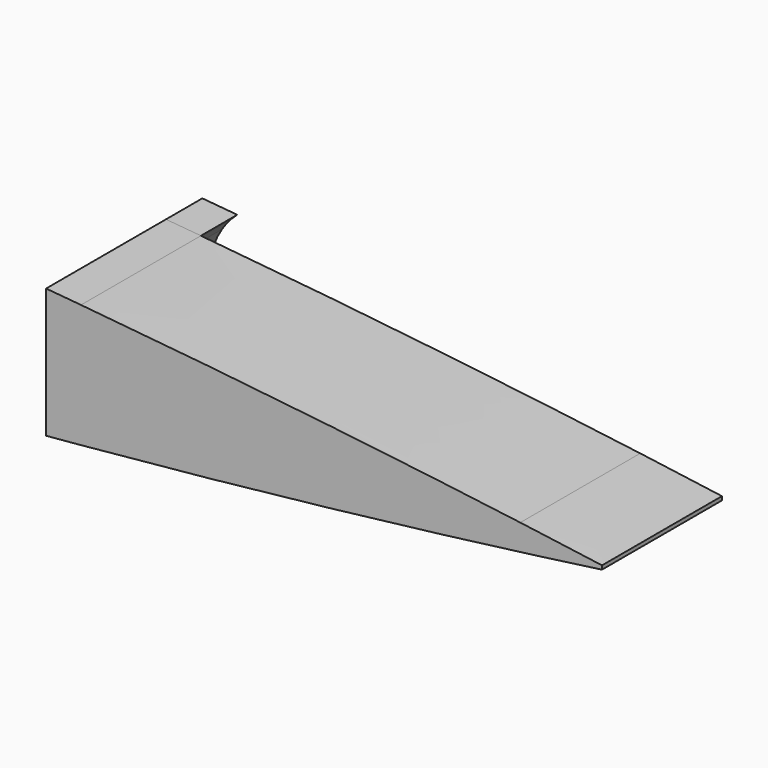
from build123d import *

# Parameters (mm, degrees)
F1_DEPTH = 82.5
F2_DEPTH = 25
F3_R     = 12.5
F4_DEPTH = 60


with BuildPart() as f1:
    # F0 (on Front) → F1 (new body)
    with BuildSketch(Plane.XZ):
        with BuildLine():
            add(Edge.make_bspline(
                [(524.024, 35.6715651167), (530.4529675183, 35.1109062879), (536.8603422789, 34.540475321), (543.2421, 33.9614)],
                knots=[0.6159550767, 0.6159550767, 0.6159550767, 0.6159550767, 0.635369827, 0.635369827, 0.635369827, 0.635369827], degree=3))
            Line((524.024, 35.6715651167), (524.024, 25.1107127602))
            add(Edge.make_bspline(
                [(524.024, 25.1107127602), (526.6770638269, 24.868020166), (530.2603237936, 24.5375720807), (533.8432643328, 24.2037227591), (534.7735361573, 24.1168150682)],
                knots=[513.3651484855, 513.3651484855, 513.3651484855, 513.3651484855, 521.3575419642, 524.1605032173, 524.1605032173, 524.1605032173, 524.1605032173], degree=3))
            ThreePointArc((534.7735361573, 24.1168150682), (538.650838246, 29.3461907199), (543.2421, 33.9614))
        make_face()
        with BuildLine():
            Line((524.024, -23.2286070743), (524.024, -35.6715651167))
            add(Edge.make_bspline(
                [(524.024, -35.6715651167), (530.4529675183, -35.1109062879), (536.8603422789, -34.540475321), (543.2421, -33.9614)],
                knots=[0.6159550767, 0.6159550767, 0.6159550767, 0.6159550767, 0.635369827, 0.635369827, 0.635369827, 0.635369827], degree=3))
            ThreePointArc((543.2421, -33.9614), (537.9689313182, -28.5343309954), (533.6796750092, -22.3004184004))
            add(Edge.make_bspline(
                [(524.024, -23.2286070743), (526.7063477836, -22.9731340758), (529.9249490386, -22.6641634275), (533.1432820941, -22.3524476401), (533.6796750092, -22.3004184004)],
                knots=[513.2741132252, 513.2741132252, 513.2741132252, 513.2741132252, 521.3575419641, 522.9742691651, 522.9742691651, 522.9742691651, 522.9742691651], degree=3))
        make_face()
        with BuildLine():
            add(Edge.make_bspline(
                [(524.024, 25.1107127602), (526.6770638269, 24.868020166), (530.2603237936, 24.5375720807), (533.8432643328, 24.2037227591), (534.7735361573, 24.1168150682)],
                knots=[513.3651484855, 513.3651484855, 513.3651484855, 513.3651484855, 521.3575419642, 524.1605032173, 524.1605032173, 524.1605032173, 524.1605032173], degree=3))
            Line((524.024, 25.1107127602), (524.024, 0))
            Line((524.024, 0), (527.7653672657, 0))
            ThreePointArc((527.7653672657, 0), (529.5529130431, 12.5572210326), (534.7735361573, 24.1168150682))
        make_face()
        with BuildLine():
            Line((524.024, 0), (524.024, -23.2286070743))
            add(Edge.make_bspline(
                [(524.024, -23.2286070743), (526.7063477836, -22.9731340758), (529.9249490386, -22.6641634275), (533.1432820941, -22.3524476401), (533.6796750092, -22.3004184004)],
                knots=[513.2741132252, 513.2741132252, 513.2741132252, 513.2741132252, 521.3575419641, 522.9742691651, 522.9742691651, 522.9742691651, 522.9742691651], degree=3))
            ThreePointArc((533.6796750092, -22.3004184004), (529.2690677016, -11.535680484), (527.7653672657, 0))
            Line((527.7653672657, 0), (524.024, 0))
        make_face()
        with BuildLine():
            add(Edge.make_bspline(
                [(543.2421, 33.9614), (549.5750436875, 33.3867540232), (562.1338476881, 32.225672374), (580.7053749717, 30.4486309004), (598.8899905971, 28.6520916952), (616.645063933, 26.8456524154), (633.9293517992, 25.0378311486), (650.7021084927, 23.2377895738), (666.924523511, 21.4542053534), (682.5583919944, 19.6948931431), (697.5675188661, 17.9689901739), (711.9166403588, 16.2843520174), (725.5723159977, 14.6495448382), (738.5025922877, 13.0722198932), (750.6773575973, 11.5611505206), (762.0679980169, 10.123355488), (772.6482697775, 8.767506964), (780.1684058461, 7.7893010713), (784.1801262556, 7.2631536294), (785.0296548206, 7.1515377434)],
                knots=[0.635369827, 0.635369827, 0.635369827, 0.635369827, 0.654636074, 0.6737293504, 0.6926255053, 0.7112999065, 0.7297277282, 0.747883428, 0.7657412837, 0.7832747177, 0.8004566202, 0.8172588362, 0.8336522425, 0.8496064603, 0.8650895564, 0.8800677295, 0.8945049966, 0.9083621399, 0.9121165786, 0.9121165786, 0.9121165786, 0.9121165786], degree=3))
            ThreePointArc((543.2421, 33.9614), (538.650838246, 29.3461907199), (534.7735361573, 24.1168150682))
            add(Edge.make_bspline(
                [(534.7735361573, 24.1168150682), (547.4888491387, 22.9289273345), (570.2810474133, 20.7234876988), (602.9514797769, 17.4132456465), (629.5721727855, 14.5753690345), (646.1150179567, 12.7470797563), (652.7777391491, 12)],
                knots=[524.1605032173, 524.1605032173, 524.1605032173, 524.1605032173, 562.4724553443, 592.8561025481, 622.6732889332, 642.7866986571, 642.7866986571, 642.7866986571, 642.7866986571], degree=3))
            Line((652.7777391491, 12), (665.973, 12))
            ThreePointArc((665.973, 12), (669.6925428199, 11.4089877382), (673.0457030707, 9.6941668684))
            add(Edge.make_bspline(
                [(673.0457030707, 9.6941668684), (678.6430527256, 9.0482316549), (693.2761814168, 7.3399638663), (715.1021603081, 4.7178028299), (732.4511827497, 2.5525104658), (740.7700852943, 1.4970109313), (741.8962423005, 1.3538186415)],
                knots=[663.1854009899, 663.1854009899, 663.1854009899, 663.1854009899, 680.0888797975, 707.3828314911, 729.1339381861, 732.5396092821, 732.5396092821, 732.5396092821, 732.5396092821], degree=3))
            add(Edge.make_bspline(
                [(741.8962423005, 1.3538186415), (746.2843670673, 1.9285048035), (754.6747553371, 3.0362373869), (766.9194584147, 4.6744667559), (776.9091256945, 6.0324501077), (782.8966080674, 6.8566568424), (785.0296548206, 7.1515377434)],
                knots=[732.5396092819, 732.5396092819, 732.5396092819, 732.5396092819, 745.8163943039, 757.9291810967, 769.6010098164, 776.0610078587, 776.0610078587, 776.0610078587, 776.0610078587], degree=3))
        make_face()
        with BuildLine():
            ThreePointArc((533.6796750092, -22.3004184004), (537.9689313182, -28.5343309954), (543.2421, -33.9614))
            add(Edge.make_bspline(
                [(543.2421, -33.9614), (549.5750436875, -33.3867540232), (562.1338476881, -32.225672374), (580.7053749717, -30.4486309004), (598.8899905971, -28.6520916952), (616.645063933, -26.8456524154), (633.9293517992, -25.0378311486), (650.7021084927, -23.2377895738), (666.924523511, -21.4542053534), (682.5583919944, -19.6948931431), (697.5675188661, -17.9689901739), (711.9166403588, -16.2843520174), (725.5723159977, -14.6495448382), (738.5025922877, -13.0722198932), (750.6773575973, -11.5611505206), (762.0679980169, -10.123355488), (772.6482697775, -8.767506964), (782.3928967751, -7.4999432572), (789.9922436278, -6.4986676858), (794.3093421293, -5.9243671687), (795.7553403022, -5.731408495)],
                knots=[0.635369827, 0.635369827, 0.635369827, 0.635369827, 0.654636074, 0.6737293504, 0.6926255053, 0.7112999065, 0.7297277282, 0.747883428, 0.7657412837, 0.7832747177, 0.8004566202, 0.8172588362, 0.8336522425, 0.8496064603, 0.8650895564, 0.8800677295, 0.8945049966, 0.9083621399, 0.921596776, 0.9284158886, 0.9284158886, 0.9284158886, 0.9284158886], degree=3))
            add(Edge.make_bspline(
                [(752.4752127939, 0), (753.3385987131, -0.1111737387), (758.2064040588, -0.7388852768), (766.9317355754, -1.8729638235), (778.4845581837, -3.3993366737), (788.0433504555, -4.682906586), (793.7449819172, -5.4572465403), (795.7553403022, -5.731408495)],
                knots=[743.2048524915, 743.2048524915, 743.2048524915, 743.2048524915, 745.816394304, 757.9291810969, 769.6010098166, 780.7760242539, 786.8629233002, 786.8629233002, 786.8629233002, 786.8629233002], degree=3))
            Line((752.4752127939, 0), (731.4902537549, 0))
            add(Edge.make_bspline(
                [(675.7749550869, -6.922548409), (680.4704196169, -6.3608211123), (694.1976504575, -4.7032327955), (712.7702276209, -2.4012449385), (726.6428498764, -0.6263462539), (731.4902537549, 0)],
                knots=[665.902054437, 665.902054437, 665.902054437, 665.902054437, 680.0888797974, 707.382831491, 722.0459285975, 722.0459285975, 722.0459285975, 722.0459285975], degree=3))
            ThreePointArc((675.7749550869, -6.922548409), (671.4924845363, -10.6552940107), (665.973, -12))
            Line((665.973, -12), (632.0462382215, -12))
            add(Edge.make_bspline(
                [(579.5327593007, -17.6845550908), (587.4225464727, -16.8640224682), (604.9318542045, -15.0134548613), (622.4325289508, -13.08262656), (632.0462382215, -12)],
                knots=[569.0591158558, 569.0591158558, 569.0591158558, 569.0591158558, 592.856102548, 621.8794937898, 621.8794937898, 621.8794937898, 621.8794937898], degree=3))
            add(Edge.make_bspline(
                [(569.024, -20), (574.601223494, -20), (579.5327593007, -17.6845550908)],
                knots=[4.7123889804, 4.7123889804, 4.7123889804, 5.1983473252, 5.1983473252, 5.1983473252], degree=2, weights=[1, 0.9706255083, 1]))
            add(Edge.make_bspline(
                [(563.3375761456, -19.3507371729), (566.1338768344, -20), (569.024, -20)],
                knots=[4.4568882152, 4.4568882152, 4.4568882152, 4.7123889804, 4.7123889804, 4.7123889804], degree=2, weights=[1, 0.9918510117, 1]))
            add(Edge.make_bspline(
                [(533.6796750092, -22.3004184004), (543.5680241797, -21.3412646258), (553.4538623678, -20.3564530629), (563.3375761456, -19.3507371729)],
                knots=[522.9742691651, 522.9742691651, 522.9742691651, 522.9742691651, 552.7784716909, 552.7784716909, 552.7784716909, 552.7784716909], degree=3))
        make_face()
        with BuildLine():
            add(Edge.make_bspline(
                [(534.7735361573, 24.1168150682), (547.4888491387, 22.9289273345), (570.2810474133, 20.7234876988), (602.9514797769, 17.4132456465), (629.5721727855, 14.5753690345), (646.1150179567, 12.7470797563), (652.7777391491, 12)],
                knots=[524.1605032173, 524.1605032173, 524.1605032173, 524.1605032173, 562.4724553443, 592.8561025481, 622.6732889332, 642.7866986571, 642.7866986571, 642.7866986571, 642.7866986571], degree=3))
            ThreePointArc((534.7735361573, 24.1168150682), (529.5529130431, 12.5572210326), (527.7653672657, 0))
            Line((527.7653672657, 0), (546.524, 0))
            add(Edge.make_bspline(
                [(591.524, 0), (591.524, 20), (569.024, 20), (546.524, 20), (546.524, 0)],
                knots=[0, 0, 0, 1.5707963268, 1.5707963268, 3.1415926536, 3.1415926536, 3.1415926536], degree=2, weights=[1, 0.7071067812, 1, 0.7071067812, 1]))
            Line((591.524, 0), (623.973, 0))
            Line((623.973, 0), (623.973, 10))
            ThreePointArc((623.973, 10), (624.5587864376, 11.4142135624), (625.973, 12))
            Line((625.973, 12), (652.7777391491, 12))
        make_face()
        with BuildLine():
            ThreePointArc((527.7653672657, 0), (529.2690677016, -11.535680484), (533.6796750092, -22.3004184004))
            add(Edge.make_bspline(
                [(533.6796750092, -22.3004184004), (543.5680241797, -21.3412646258), (553.4538623678, -20.3564530629), (563.3375761456, -19.3507371729)],
                knots=[522.9742691651, 522.9742691651, 522.9742691651, 522.9742691651, 552.7784716909, 552.7784716909, 552.7784716909, 552.7784716909], degree=3))
            add(Edge.make_bspline(
                [(546.524, 0), (546.524, -15.4468544374), (563.3375761456, -19.3507371729)],
                knots=[3.1415926536, 3.1415926536, 3.1415926536, 4.4568882152, 4.4568882152, 4.4568882152], degree=2, weights=[1, 0.7914322299, 1]))
            Line((546.524, 0), (527.7653672657, 0))
        make_face()
        with BuildLine():
            add(Edge.make_bspline(
                [(785.0296548206, 7.1515377434), (787.174768668, 6.8697005072), (792.0785180819, 6.2224623401), (799.2875794028, 5.2606805783), (806.398007937, 4.3017234095), (812.5937368846, 3.4579115596), (817.8623783077, 2.7342517017), (822.1845332462, 2.1365671069), (825.5717903187, 1.6654782983), (827.9484571682, 1.33323589), (829.4727060537, 1.1198422864), (829.8586880275, 1.0656429389), (830, 1.0458)],
                knots=[0.9121165786, 0.9121165786, 0.9121165786, 0.9121165786, 0.921596776, 0.9341612481, 0.9460018444, 0.9570561288, 0.9672492741, 0.9764880356, 0.9846490394, 0.9915545746, 0.9969080429, 1, 1, 1, 1], degree=3))
            add(Edge.make_bspline(
                [(741.8962423005, 1.3538186415), (746.2843670673, 1.9285048035), (754.6747553371, 3.0362373869), (766.9194584147, 4.6744667559), (776.9091256945, 6.0324501077), (782.8966080674, 6.8566568424), (785.0296548206, 7.1515377434)],
                knots=[732.5396092819, 732.5396092819, 732.5396092819, 732.5396092819, 745.8163943039, 757.9291810967, 769.6010098164, 776.0610078587, 776.0610078587, 776.0610078587, 776.0610078587], degree=3))
            add(Edge.make_bspline(
                [(741.8962423005, 1.3538186415), (745.4229300003, 0.9053958333), (748.9492417496, 0.4540210524), (752.4752127939, 0)],
                knots=[732.5396092821, 732.5396092821, 732.5396092821, 732.5396092821, 743.2048524915, 743.2048524915, 743.2048524915, 743.2048524915], degree=3))
            Line((752.4752127939, 0), (830, 0))
            Line((830, 0), (830, 1.0458))
        make_face()
        with BuildLine():
            add(Edge.make_bspline(
                [(752.4752127939, 0), (753.3385987131, -0.1111737387), (758.2064040588, -0.7388852768), (766.9317355754, -1.8729638235), (778.4845581837, -3.3993366737), (788.0433504555, -4.682906586), (793.7449819172, -5.4572465403), (795.7553403022, -5.731408495)],
                knots=[743.2048524915, 743.2048524915, 743.2048524915, 743.2048524915, 745.816394304, 757.9291810969, 769.6010098166, 780.7760242539, 786.8629233002, 786.8629233002, 786.8629233002, 786.8629233002], degree=3))
            add(Edge.make_bspline(
                [(795.7553403022, -5.731408495), (796.9736482838, -5.568833537), (800.6549707765, -5.0762655667), (806.398007937, -4.3017234095), (812.5937368846, -3.4579115596), (817.8623783077, -2.7342517017), (822.1845332462, -2.1365671069), (825.5717903187, -1.6654782983), (827.9484571682, -1.33323589), (829.4727060537, -1.1198422864), (829.8586880275, -1.0656429389), (830, -1.0458)],
                knots=[0.9284158886, 0.9284158886, 0.9284158886, 0.9284158886, 0.9341612481, 0.9460018444, 0.9570561288, 0.9672492741, 0.9764880356, 0.9846490394, 0.9915545746, 0.9969080429, 1, 1, 1, 1], degree=3))
            Line((830, -1.0458), (830, 0))
            Line((830, 0), (752.4752127939, 0))
        make_face()
        with BuildLine():
            Line((665.973, 12), (652.7777391491, 12))
            add(Edge.make_bspline(
                [(652.7777391491, 12), (655.762922623, 11.6652763822), (660.161514663, 11.1688961032), (664.5595773708, 10.6678568096), (665.973, 10.5063520034)],
                knots=[642.7866986571, 642.7866986571, 642.7866986571, 642.7866986571, 651.7983646979, 656.0662217526, 656.0662217526, 656.0662217526, 656.0662217526], degree=3))
            Line((665.973, 10.5063520034), (665.973, 12))
        make_face()
        with BuildLine():
            add(Edge.make_bspline(
                [(652.7777391491, 12), (655.762922623, 11.6652763822), (660.161514663, 11.1688961032), (664.5595773708, 10.6678568096), (665.973, 10.5063520034)],
                knots=[642.7866986571, 642.7866986571, 642.7866986571, 642.7866986571, 651.7983646979, 656.0662217526, 656.0662217526, 656.0662217526, 656.0662217526], degree=3))
            Line((652.7777391491, 12), (625.973, 12))
            ThreePointArc((625.973, 12), (624.5587864376, 11.4142135624), (623.973, 10))
            Line((623.973, 10), (623.973, 0))
            Line((623.973, 0), (665.973, 0))
            Line((665.973, 0), (665.973, 10.5063520034))
        make_face()
        with BuildLine():
            add(Edge.make_bspline(
                [(546.524, 0), (546.524, -15.4468544374), (563.3375761456, -19.3507371729)],
                knots=[3.1415926536, 3.1415926536, 3.1415926536, 4.4568882152, 4.4568882152, 4.4568882152], degree=2, weights=[1, 0.7914322299, 1]))
            add(Edge.make_bspline(
                [(563.3375761456, -19.3507371729), (566.5523093603, -19.0236224518), (571.9509432397, -18.4705327095), (577.3489807289, -17.911666611), (579.5327593007, -17.6845550908)],
                knots=[552.7784716909, 552.7784716909, 552.7784716909, 552.7784716909, 562.4724553442, 569.0591158558, 569.0591158558, 569.0591158558, 569.0591158558], degree=3))
            add(Edge.make_bspline(
                [(579.5327593007, -17.6845550908), (591.524, -12.0544515447), (591.524, 0)],
                knots=[5.1983473252, 5.1983473252, 5.1983473252, 6.2831853072, 6.2831853072, 6.2831853072], degree=2, weights=[1, 0.8564624828, 1]))
            Line((591.524, 0), (546.524, 0))
        make_face()
        with BuildLine():
            add(Edge.make_bspline(
                [(563.3375761456, -19.3507371729), (566.5523093603, -19.0236224518), (571.9509432397, -18.4705327095), (577.3489807289, -17.911666611), (579.5327593007, -17.6845550908)],
                knots=[552.7784716909, 552.7784716909, 552.7784716909, 552.7784716909, 562.4724553442, 569.0591158558, 569.0591158558, 569.0591158558, 569.0591158558], degree=3))
            add(Edge.make_bspline(
                [(563.3375761456, -19.3507371729), (566.1338768344, -20), (569.024, -20)],
                knots=[4.4568882152, 4.4568882152, 4.4568882152, 4.7123889804, 4.7123889804, 4.7123889804], degree=2, weights=[1, 0.9918510117, 1]))
            add(Edge.make_bspline(
                [(569.024, -20), (574.601223494, -20), (579.5327593007, -17.6845550908)],
                knots=[4.7123889804, 4.7123889804, 4.7123889804, 5.1983473252, 5.1983473252, 5.1983473252], degree=2, weights=[1, 0.9706255083, 1]))
        make_face()
        with BuildLine():
            add(Edge.make_bspline(
                [(731.4902537549, 0), (733.8334453003, 0.3027701597), (737.3022307159, 0.7531116765), (740.7706302145, 1.2064040341), (741.8962423005, 1.3538186415)],
                knots=[722.0459285975, 722.0459285975, 722.0459285975, 722.0459285975, 729.1339381859, 732.5396092819, 732.5396092819, 732.5396092819, 732.5396092819], degree=3))
            add(Edge.make_bspline(
                [(673.0457030707, 9.6941668684), (678.6430527256, 9.0482316549), (693.2761814168, 7.3399638663), (715.1021603081, 4.7178028299), (732.4511827497, 2.5525104658), (740.7700852943, 1.4970109313), (741.8962423005, 1.3538186415)],
                knots=[663.1854009899, 663.1854009899, 663.1854009899, 663.1854009899, 680.0888797975, 707.3828314911, 729.1339381861, 732.5396092821, 732.5396092821, 732.5396092821, 732.5396092821], degree=3))
            ThreePointArc((673.0457030707, 9.6941668684), (676.6704865471, 5.4372586453), (677.973, 0))
            Line((677.973, 0), (731.4902537549, 0))
        make_face()
        with BuildLine():
            add(Edge.make_bspline(
                [(741.8962423005, 1.3538186415), (745.4229300003, 0.9053958333), (748.9492417496, 0.4540210524), (752.4752127939, 0)],
                knots=[732.5396092821, 732.5396092821, 732.5396092821, 732.5396092821, 743.2048524915, 743.2048524915, 743.2048524915, 743.2048524915], degree=3))
            add(Edge.make_bspline(
                [(731.4902537549, 0), (733.8334453003, 0.3027701597), (737.3022307159, 0.7531116765), (740.7706302145, 1.2064040341), (741.8962423005, 1.3538186415)],
                knots=[722.0459285975, 722.0459285975, 722.0459285975, 722.0459285975, 729.1339381859, 732.5396092819, 732.5396092819, 732.5396092819, 732.5396092819], degree=3))
            Line((731.4902537549, 0), (752.4752127939, 0))
        make_face()
        with BuildLine():
            add(Edge.make_bspline(
                [(591.524, 0), (591.524, 20), (569.024, 20), (546.524, 20), (546.524, 0)],
                knots=[0, 0, 0, 1.5707963268, 1.5707963268, 3.1415926536, 3.1415926536, 3.1415926536], degree=2, weights=[1, 0.7071067812, 1, 0.7071067812, 1]))
            Line((546.524, 0), (591.524, 0))
        make_face()
        with BuildLine():
            Line((665.973, 12), (665.973, 10.5063520034))
            add(Edge.make_bspline(
                [(665.973, 10.5063520034), (668.3307193205, 10.2369470894), (670.6882868311, 9.9662131504), (673.0457030707, 9.6941668684)],
                knots=[656.0662217526, 656.0662217526, 656.0662217526, 656.0662217526, 663.1854009899, 663.1854009899, 663.1854009899, 663.1854009899], degree=3))
            ThreePointArc((673.0457030707, 9.6941668684), (669.6925428199, 11.4089877382), (665.973, 12))
        make_face()
        with BuildLine():
            add(Edge.make_bspline(
                [(665.973, 10.5063520034), (668.3307193205, 10.2369470894), (670.6882868311, 9.9662131504), (673.0457030707, 9.6941668684)],
                knots=[656.0662217526, 656.0662217526, 656.0662217526, 656.0662217526, 663.1854009899, 663.1854009899, 663.1854009899, 663.1854009899], degree=3))
            Line((665.973, 10.5063520034), (665.973, 0))
            Line((665.973, 0), (677.973, 0))
            ThreePointArc((677.973, 0), (676.6704865471, 5.4372586453), (673.0457030707, 9.6941668684))
        make_face()
        with BuildLine():
            add(Edge.make_bspline(
                [(579.5327593007, -17.6845550908), (591.524, -12.0544515447), (591.524, 0)],
                knots=[5.1983473252, 5.1983473252, 5.1983473252, 6.2831853072, 6.2831853072, 6.2831853072], degree=2, weights=[1, 0.8564624828, 1]))
            add(Edge.make_bspline(
                [(579.5327593007, -17.6845550908), (587.4225464727, -16.8640224682), (604.9318542045, -15.0134548613), (622.4325289508, -13.08262656), (632.0462382215, -12)],
                knots=[569.0591158558, 569.0591158558, 569.0591158558, 569.0591158558, 592.856102548, 621.8794937898, 621.8794937898, 621.8794937898, 621.8794937898], degree=3))
            Line((632.0462382215, -12), (625.973, -12))
            ThreePointArc((625.973, -12), (624.5587864376, -11.4142135624), (623.973, -10))
            Line((623.973, -10), (623.973, 0))
            Line((623.973, 0), (591.524, 0))
        make_face()
        with BuildLine():
            add(Edge.make_bspline(
                [(675.7749550869, -6.922548409), (680.4704196169, -6.3608211123), (694.1976504575, -4.7032327955), (712.7702276209, -2.4012449385), (726.6428498764, -0.6263462539), (731.4902537549, 0)],
                knots=[665.902054437, 665.902054437, 665.902054437, 665.902054437, 680.0888797974, 707.382831491, 722.0459285975, 722.0459285975, 722.0459285975, 722.0459285975], degree=3))
            Line((731.4902537549, 0), (677.973, 0))
            ThreePointArc((677.973, 0), (677.4102955947, -3.6315657062), (675.7749550869, -6.922548409))
        make_face()
        with BuildLine():
            Line((665.973, -8.0874938306), (665.973, 0))
            Line((665.973, 0), (623.973, 0))
            Line((623.973, 0), (623.973, -10))
            ThreePointArc((623.973, -10), (624.5587864376, -11.4142135624), (625.973, -12))
            Line((625.973, -12), (632.0462382215, -12))
            add(Edge.make_bspline(
                [(632.0462382215, -12), (632.3091749564, -11.9703899624), (642.2194339984, -10.8537488755), (653.528780869, -9.5529086768), (664.5718113348, -8.2529185042), (665.973, -8.0874938306)],
                knots=[621.8794937898, 621.8794937898, 621.8794937898, 621.8794937898, 622.6732889331, 651.7983646977, 656.0311218622, 656.0311218622, 656.0311218622, 656.0311218622], degree=3))
        make_face()
        with BuildLine():
            Line((677.973, 0), (665.973, 0))
            Line((665.973, 0), (665.973, -8.0874938306))
            add(Edge.make_bspline(
                [(665.973, -8.0874938306), (669.2406192612, -7.7017179081), (672.5079370891, -7.3133879471), (675.7749550869, -6.922548409)],
                knots=[656.0311218622, 656.0311218622, 656.0311218622, 656.0311218622, 665.902054437, 665.902054437, 665.902054437, 665.902054437], degree=3))
            ThreePointArc((675.7749550869, -6.922548409), (677.4102955947, -3.6315657062), (677.973, 0))
        make_face()
        with BuildLine():
            add(Edge.make_bspline(
                [(632.0462382215, -12), (632.3091749564, -11.9703899624), (642.2194339984, -10.8537488755), (653.528780869, -9.5529086768), (664.5718113348, -8.2529185042), (665.973, -8.0874938306)],
                knots=[621.8794937898, 621.8794937898, 621.8794937898, 621.8794937898, 622.6732889331, 651.7983646977, 656.0311218622, 656.0311218622, 656.0311218622, 656.0311218622], degree=3))
            Line((632.0462382215, -12), (665.973, -12))
            Line((665.973, -12), (665.973, -8.0874938306))
        make_face()
        with BuildLine():
            ThreePointArc((665.973, -12), (671.4924845363, -10.6552940107), (675.7749550869, -6.922548409))
            add(Edge.make_bspline(
                [(665.973, -8.0874938306), (669.2406192612, -7.7017179081), (672.5079370891, -7.3133879471), (675.7749550869, -6.922548409)],
                knots=[656.0311218622, 656.0311218622, 656.0311218622, 656.0311218622, 665.902054437, 665.902054437, 665.902054437, 665.902054437], degree=3))
            Line((665.973, -8.0874938306), (665.973, -12))
        make_face()
    extrude(amount=F1_DEPTH)

    # F0 (on Front) → F2 (join)
    with BuildSketch(Plane.XZ):
        with BuildLine():
            add(Edge.make_bspline(
                [(524.024, 35.6715651167), (530.4529675183, 35.1109062879), (536.8603422789, 34.540475321), (543.2421, 33.9614)],
                knots=[0.6159550767, 0.6159550767, 0.6159550767, 0.6159550767, 0.635369827, 0.635369827, 0.635369827, 0.635369827], degree=3))
            Line((524.024, 35.6715651167), (524.024, 25.1107127602))
            add(Edge.make_bspline(
                [(524.024, 25.1107127602), (526.6770638269, 24.868020166), (530.2603237936, 24.5375720807), (533.8432643328, 24.2037227591), (534.7735361573, 24.1168150682)],
                knots=[513.3651484855, 513.3651484855, 513.3651484855, 513.3651484855, 521.3575419642, 524.1605032173, 524.1605032173, 524.1605032173, 524.1605032173], degree=3))
            ThreePointArc((534.7735361573, 24.1168150682), (538.650838246, 29.3461907199), (543.2421, 33.9614))
        make_face()
        with BuildLine():
            Line((524.024, -23.2286070743), (524.024, -35.6715651167))
            add(Edge.make_bspline(
                [(524.024, -35.6715651167), (530.4529675183, -35.1109062879), (536.8603422789, -34.540475321), (543.2421, -33.9614)],
                knots=[0.6159550767, 0.6159550767, 0.6159550767, 0.6159550767, 0.635369827, 0.635369827, 0.635369827, 0.635369827], degree=3))
            ThreePointArc((543.2421, -33.9614), (537.9689313182, -28.5343309954), (533.6796750092, -22.3004184004))
            add(Edge.make_bspline(
                [(524.024, -23.2286070743), (526.7063477836, -22.9731340758), (529.9249490386, -22.6641634275), (533.1432820941, -22.3524476401), (533.6796750092, -22.3004184004)],
                knots=[513.2741132252, 513.2741132252, 513.2741132252, 513.2741132252, 521.3575419641, 522.9742691651, 522.9742691651, 522.9742691651, 522.9742691651], degree=3))
        make_face()
        with BuildLine():
            add(Edge.make_bspline(
                [(524.024, 25.1107127602), (526.6770638269, 24.868020166), (530.2603237936, 24.5375720807), (533.8432643328, 24.2037227591), (534.7735361573, 24.1168150682)],
                knots=[513.3651484855, 513.3651484855, 513.3651484855, 513.3651484855, 521.3575419642, 524.1605032173, 524.1605032173, 524.1605032173, 524.1605032173], degree=3))
            Line((524.024, 25.1107127602), (524.024, 0))
            Line((524.024, 0), (527.7653672657, 0))
            ThreePointArc((527.7653672657, 0), (529.5529130431, 12.5572210326), (534.7735361573, 24.1168150682))
        make_face()
        with BuildLine():
            Line((524.024, 0), (524.024, -23.2286070743))
            add(Edge.make_bspline(
                [(524.024, -23.2286070743), (526.7063477836, -22.9731340758), (529.9249490386, -22.6641634275), (533.1432820941, -22.3524476401), (533.6796750092, -22.3004184004)],
                knots=[513.2741132252, 513.2741132252, 513.2741132252, 513.2741132252, 521.3575419641, 522.9742691651, 522.9742691651, 522.9742691651, 522.9742691651], degree=3))
            ThreePointArc((533.6796750092, -22.3004184004), (529.2690677016, -11.535680484), (527.7653672657, 0))
            Line((527.7653672657, 0), (524.024, 0))
        make_face()
    extrude(amount=-F2_DEPTH)

    # F3 (on face) → F4 (cut)
    with BuildSketch(Plane.XZ):
        with Locations((572.7653672657, 0)):
            Circle(F3_R)
    extrude(amount=F4_DEPTH, mode=Mode.SUBTRACT)


solid = f1.part
